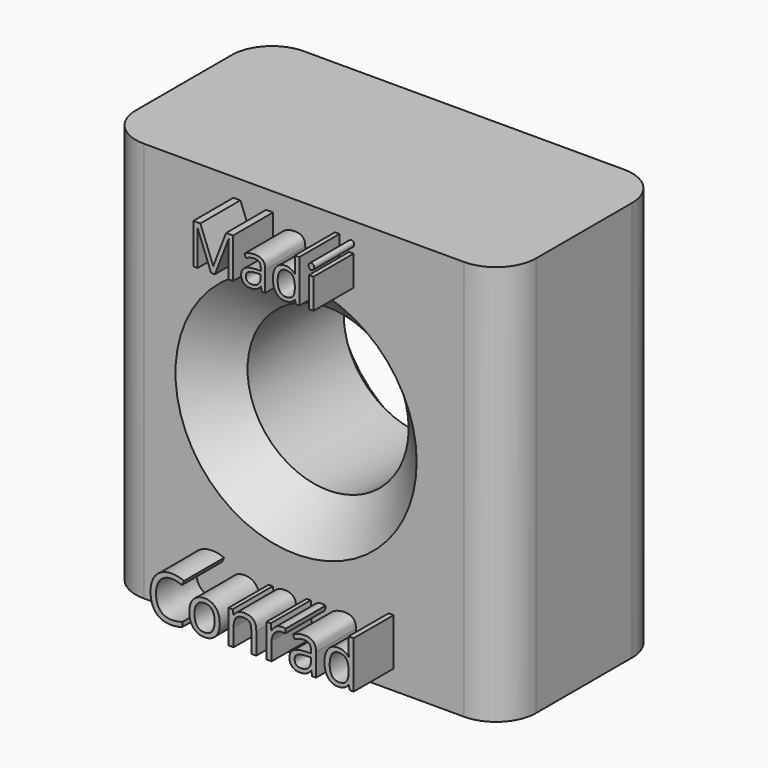
from build123d import *

# Parameters (mm, degrees)
F0_W           = 25.4
F0_H           = 25.4
F0_R           = 5.1109259981
F1_DEPTH       = 12.7
F2_TEXT_SIZE   = 3.5639140858
F2_TEXT_SIZE_2 = 3.9294439678
F3_DEPTH       = 3.175
F4_R           = 2.54
F5_R           = 2.54
F6_SIZE        = 2.54


# Not quite as in the source:
# - Text() gives the source's letters only with a copy of the font that has no kerning and outlines rounded to 1/6400 em; it was checked with that copy


with BuildPart() as f1:
    # F0 (on Front) → F1 (new body)
    with BuildSketch(Plane.XZ):
        with Locations((20.2183973372, -0.5587999105)):
            Rectangle(F0_W, F0_H)
        with Locations((19.719818607, 0)):
            Circle(F0_R, mode=Mode.SUBTRACT)
    extrude(amount=F1_DEPTH)

    # F2 (on face) → F3 (join)
    with BuildSketch(Plane.XZ.offset(12.7)):
        with Locations((15.3932459652, 8.4253149107)):
            Text('Madi', F2_TEXT_SIZE, font='Open Sans', text_align=(TextAlign.LEFT, TextAlign.BOTTOM))
        with Locations((12.7873234451, -12.0188770816)):
            Text('Conrad', F2_TEXT_SIZE_2, font='Open Sans', text_align=(TextAlign.LEFT, TextAlign.BOTTOM))
    extrude(amount=F3_DEPTH)

    # F4
    f4_edges = [f1.edges().sort_by_distance(p)[0] for p in [
        (32.918397, -12.7, -0.5588),
    ]]
    fillet(f4_edges, radius=F4_R)

    # F5
    f5_edges = [f1.edges().sort_by_distance(p)[0] for p in [
        (32.918397, 0, -0.5588),
        (7.518397, 0, -0.5588),
        (7.518397, -12.7, -0.5588),
    ]]
    fillet(f5_edges, radius=F5_R)

    # F6
    f6_edges = [f1.edges().sort_by_distance(p)[0] for p in [
        (14.608893, -12.7, 0),
        (14.608893, 0, 0),
    ]]
    chamfer(f6_edges, length=F6_SIZE)


solid = f1.part
